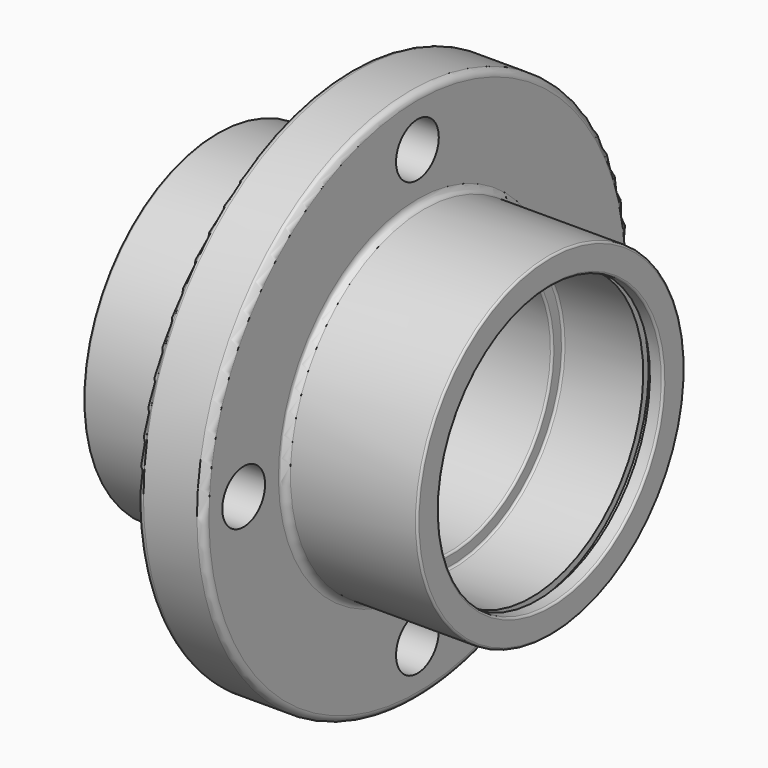
from build123d import *

# Parameters (mm, degrees)
F2_R     = 0.3
F3_R     = 1
F4_R     = 4
F5_DEPTH = 30.001


with BuildPart() as f1:
    # F0 (on Front) → F1 (revolve)
    with BuildSketch(Plane.XZ):
        Polygon((0, 25), (0, 21), (2, 21), (2, 22), (3, 22), (3, 21), (15, 21), (15, 19), (35, 19), (35, 21), (47, 21), (47, 22), (48, 22), (48, 21), (50, 21), (50, 25), (30, 25), (30, 40), (20, 40), (20, 25), align=None)
    revolve(axis=Axis((26.2251488414, 0, 0), (1, 0, 0)))

    # F2
    f2_edges = [f1.edges().sort_by_distance(p)[0] for p in [
        (15, 0, -21),
        (0, 0, -21),
        (15, 0, -19),
        (35, 0, -21),
        (0, 0, -25),
        (35, 0, -19),
        (50, 0, -21),
        (50, 0, -25),
    ]]
    fillet(f2_edges, radius=F2_R)

    # F3
    f3_edges = [f1.edges().sort_by_distance(p)[0] for p in [
        (30, 0, -25),
        (20, 0, -40),
        (20, 0, -25),
        (30, 0, -40),
    ]]
    fillet(f3_edges, radius=F3_R)

    # F4 (on face) → F5 (cut, through all)
    with BuildSketch(Plane.YZ.offset(30)):
        with Locations((0, 32.5)):
            Circle(F4_R)
        with Locations((-32.5, 0)):
            Circle(F4_R)
        with Locations((0, -32.5)):
            Circle(F4_R)
        with Locations((32.5, 0)):
            Circle(F4_R)
    extrude(amount=-F5_DEPTH, mode=Mode.SUBTRACT)


solid = f1.part
